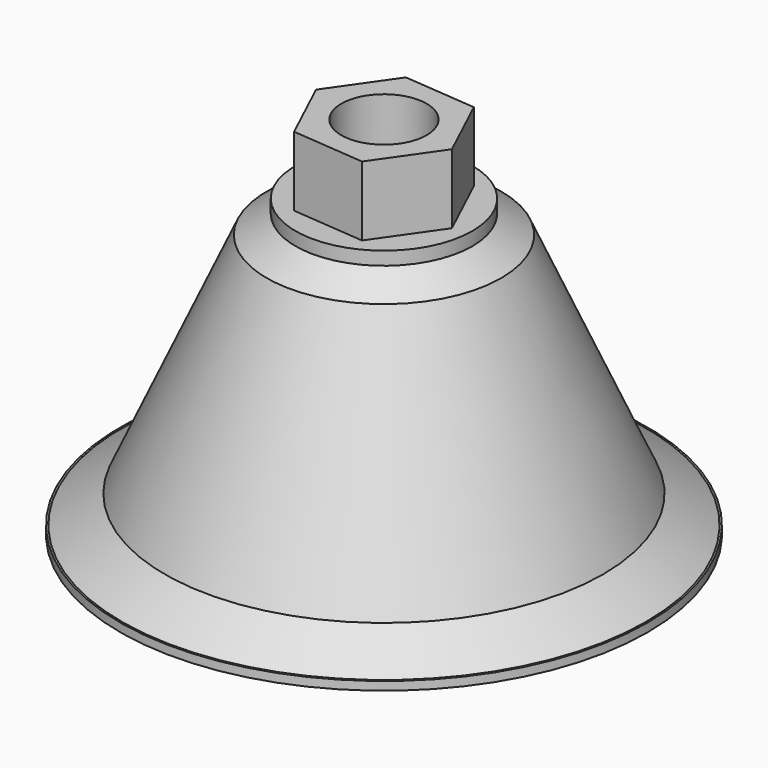
from build123d import *

# Parameters (mm, degrees)
F4_DEPTH    = 13
F5_R        = 7
F6_DEPTH    = 15
F7_R        = 14.5
F8_DEPTH    = 1.6
F9_S5_R     = 14.5
F9_T6_DEPTH = 29
F10_SIZE    = 5


# Not quite as in the source:
# - a fillet or chamfer that OpenCascade refuses, or shapes differently, is made with other operations: its cross-section is extruded or revolved along the edge and cut away or added
# - a feature names something its author has since deleted; it is built from what else it names


with BuildPart() as f2:
    # F0 (on Front) → F2 (revolve)
    with BuildSketch(Plane.XZ):
        Polygon((17.6, 24.4003517207), (0, 24.4003517207), (0, 23.0003517207), (14, 23.0003517207), (33.795146799, -22.8053483963), (43.2849223453, -22.5459427606), (43.2849223453, -21.1459427606), (37.9849223453, -21.1459427606), align=None)
    revolve(axis=Axis((0, 0, 12.0206931606), (0, 0, -1)))

    # F3 (on face) → F4 (join)
    with BuildSketch(Plane.XY.offset(24.4003517207)):
        Polygon((-11.9566419536, 1.0191727989), (-6.8609505115, -9.8451692763), (5.0956914421, -10.8643420752), (11.9566419536, -1.0191727989), (6.8609505115, 9.8451692763), (-5.0956914421, 10.8643420752), align=None)
    extrude(amount=F4_DEPTH)

    # F5 (on face) → F6 (cut)
    with BuildSketch(Plane.XY.offset(37.4003517207)):
        Circle(F5_R)
    extrude(amount=-F6_DEPTH, mode=Mode.SUBTRACT)

    # F7 (on face) → F8 (join)
    with BuildSketch(Plane.XY.offset(24.4003517207)):
        Circle(F7_R)
    extrude(amount=F8_DEPTH)

    # F9: chamfer of 4 on 1 edges, made by hand


with BuildPart() as f9_tool2:
    # F9_s3 → F9_t4 (revolve)
    with BuildSketch(Plane.XZ):
        Polygon((19.2340619114, 20.749346151), (13.6, 24.4003517207), (17.6, 24.4003517207), align=None)
    revolve(axis=Axis((0, 0, 24.4003517207), (0, 0, -1)))

    # F9_s5 → F9_t6 (cut, symmetric)
    with BuildSketch(Plane.XY.offset(22.6)):
        Circle(F9_S5_R)
    extrude(amount=F9_T6_DEPTH, both=True, mode=Mode.SUBTRACT)


with BuildPart() as f2_1:
    add(f2.part)

    # F9_t1: cut F9_tool2
    add(f9_tool2.part, mode=Mode.SUBTRACT)

    # F10
    f10_edges = [f2_1.edges().sort_by_distance(p)[0] for p in [
        (-37.984922, 0, -21.145943),
    ]]
    chamfer(f10_edges, length=F10_SIZE)


solid = f2_1.part
